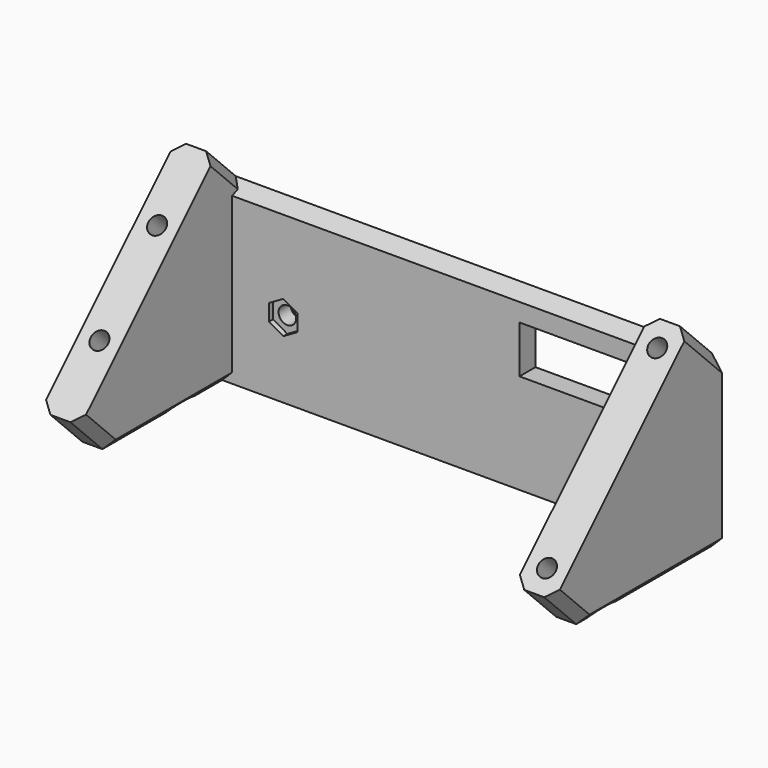
from build123d import *

# Parameters (mm, degrees)
F2_DEPTH      = 4
F5_DEPTH      = 49.55
F5_DEPTH_BACK = 53.25
F6_R          = 3.25
F6_R_2        = 1.75
F7_DEPTH      = 35.314708499
F8_DEPTH      = 5
F9_R          = 1.75
F9_W          = 23
F9_H          = 9.5
F10_DEPTH     = 4.001
F11_DEPTH     = 1
F12_T1_DEPTH  = 21.6004404508
F12_T3_DEPTH  = 86.8
F12_T5_DEPTH  = 21.6004404508
F12_T7_DEPTH  = 44.2278574488
F12_T9_DEPTH  = 35.0844914729
F12_T14_DEPTH = 15.9435862014
F12_T19_DEPTH = 15.9435862014
F12_T25_DEPTH = 98.9490097203
F12_S28_R     = 3.25
F12_T29_DEPTH = 51
F12_T32_DEPTH = 10.8002202254
F12_T39_DEPTH = 10.8002202254
F12_T43_DEPTH = 98.9490097203


# Not quite as in the source:
# - a fillet or chamfer that OpenCascade refuses, or shapes differently, is made with other operations: its cross-section is extruded or revolved along the edge and cut away or added


with BuildPart() as f2:
    # F0 (on Right) → F2 (new body, symmetric)
    with BuildSketch(Plane.YZ):
        Polygon((-8, 41.941125497), (-24.9705627485, 24.9705627485), (-41.941125497, 8), (-33.941125497, 0), (-4, 0), (-4, 37.941125497), align=None)
    extrude(amount=F2_DEPTH, both=True)


with BuildPart() as f3_1:
    # F3: copy of F2
    add(f2.part.moved(Location((-49.25, 0, 0))))


with BuildPart() as f2_1:
    # F4: moved
    add(f2.part.moved(Location((45.55, 0, 0))))


    add(f3_1.part)  # F5 merges F3_1
    # F0 (on Right) → F5 (join, two sides)
    with BuildSketch(Plane.YZ) as f5_sk:
        Polygon((0, 33.941125497), (-4, 37.941125497), (-4, 0), (0, 0), align=None)
    extrude(amount=F5_DEPTH)
    extrude(f5_sk.sketch, amount=-F5_DEPTH_BACK)

    # F6 (on line) → F7 (cut, through all)
    with BuildSketch(Plane(origin=(0, -24.9705627485, 24.9705627485), x_dir=(1, 0, 0), z_dir=(0, -0.7071067812, 0.7071067812))):
        with Locations((-49.25, 10.2)):
            Circle(F6_R)
        with Locations((-49.25, 10.2)):
            Circle(F6_R_2, mode=Mode.SUBTRACT)
        with Locations((-49.25, 10.2)):
            Circle(F6_R_2)
        with Locations((-49.25, -10.2)):
            Circle(F6_R)
        with Locations((-49.25, -10.2)):
            Circle(F6_R_2, mode=Mode.SUBTRACT)
        with Locations((-49.25, -10.2)):
            Circle(F6_R_2)
        with Locations((45.55, 19.5)):
            Circle(F6_R)
        with Locations((45.55, 19.5)):
            Circle(F6_R_2, mode=Mode.SUBTRACT)
        with Locations((45.55, 19.5)):
            Circle(F6_R_2)
        with Locations((45.55, -19.5)):
            Circle(F6_R)
        with Locations((45.55, -19.5)):
            Circle(F6_R_2, mode=Mode.SUBTRACT)
        with Locations((45.55, -19.5)):
            Circle(F6_R_2)
    extrude(amount=-F7_DEPTH, mode=Mode.SUBTRACT)

    # F6 (on line) → F8 (join)
    with BuildSketch(Plane(origin=(0, -24.9705627485, 24.9705627485), x_dir=(1, 0, 0), z_dir=(0, -0.7071067812, 0.7071067812))):
        with Locations((45.55, -19.5)):
            Circle(F6_R)
        with Locations((45.55, -19.5)):
            Circle(F6_R_2, mode=Mode.SUBTRACT)
        with Locations((45.55, 19.5)):
            Circle(F6_R)
        with Locations((45.55, 19.5)):
            Circle(F6_R_2, mode=Mode.SUBTRACT)
        with Locations((-49.25, 10.2)):
            Circle(F6_R)
        with Locations((-49.25, 10.2)):
            Circle(F6_R_2, mode=Mode.SUBTRACT)
        with Locations((-49.25, -10.2)):
            Circle(F6_R)
        with Locations((-49.25, -10.2)):
            Circle(F6_R_2, mode=Mode.SUBTRACT)
    extrude(amount=-F8_DEPTH)

    # F9 (on face) → F10 (cut, through all)
    with BuildSketch(Plane.XZ.offset(4)):
        with Locations((-35, 15)):
            Circle(F9_R)
        with Locations((35, 15)):
            Circle(F9_R)
        with Locations((23.75, 24.75)):
            Rectangle(F9_W, F9_H)
    extrude(amount=-F10_DEPTH, mode=Mode.SUBTRACT)

    # F9 (on face) → F11 (cut)
    with BuildSketch(Plane.XZ.offset(4)):
        Polygon((-32.15, 13.3545517328), (-32.15, 16.6454482672), (-35, 18.2908965344), (-37.85, 16.6454482672), (-37.85, 13.3545517328), (-35, 11.7091034656), align=None)
        with Locations((-35, 15)):
            Circle(F9_R, mode=Mode.SUBTRACT)
        Polygon((37.85, 13.3545517328), (37.85, 16.6454482672), (35, 18.2908965344), (32.15, 16.6454482672), (32.15, 13.3545517328), (35, 11.7091034656), align=None)
        with Locations((35, 15)):
            Circle(F9_R, mode=Mode.SUBTRACT)
    extrude(amount=-F11_DEPTH, mode=Mode.SUBTRACT)

    # F12: chamfer of 2 on 13 edges, made by hand

    # F12_s2 → F12_t1 (cut)
    with BuildSketch(Plane(origin=(0, -28.6074717082, 28.6074717082), x_dir=(1, 0, 0), z_dir=(0, 0.7071067812, -0.7071067812))):
        Polygon((47.55, -24), (49.55, -22), (49.55, -24), align=None)
        Polygon((-53.25, 22), (-51.25, 24), (-53.25, 24), align=None)
        Polygon((-45.25, 22), (-47.25, 24), (-45.25, 24), align=None)
        Polygon((41.55, 22), (43.55, 24), (41.55, 24), align=None)
        Polygon((49.55, 22), (47.55, 24), (49.55, 24), align=None)
    extrude(amount=F12_T1_DEPTH, mode=Mode.SUBTRACT)

    # F12_s4 → F12_t3 (cut)
    with BuildSketch(Plane.YZ.offset(-45.25)):
        Polygon((-0.5857864376, 34.5269119346), (-4, 33.1126983722), (-4, 37.941125497), align=None)
    extrude(amount=F12_T3_DEPTH, mode=Mode.SUBTRACT)

    # F12_s6 → F12_t5 (cut)
    with BuildSketch(Plane(origin=(0, -13.3336537888, 13.3336537888), x_dir=(1, 0, 0), z_dir=(0, -0.7071067812, 0.7071067812))):
        Polygon((-51.25, 24), (-53.25, 22), (-53.25, 24), align=None)
    extrude(amount=F12_T5_DEPTH, mode=Mode.SUBTRACT)

    # F12_s8 → F12_t7 (cut)
    with BuildSketch(Plane.XZ.offset(-5.1433659759)):
        Polygon((-53.25, 2), (-51.25, 0), (-53.25, 0), align=None)
        Polygon((49.55, 2), (47.55, 0), (49.55, 0), align=None)
    extrude(amount=F12_T7_DEPTH, mode=Mode.SUBTRACT)

    # F12_s10 → F12_t9 (cut)
    with BuildSketch(Plane.XZ.offset(4)):
        Polygon((-45.25, 2), (-47.25, 0), (-45.25, 0), align=None)
        Polygon((41.55, 2), (43.55, 0), (41.55, 0), align=None)
    extrude(amount=F12_T9_DEPTH, mode=Mode.SUBTRACT)


with BuildPart() as f12_tool12:
    # F12_s13 → F12_t14 (new body)
    with BuildSketch(Plane(origin=(0, -17.3336537888, 17.3336537888), x_dir=(1, 0, 0), z_dir=(0, -0.7071067812, 0.7071067812))):
        Polygon((-47.25, 24), (-45.25, 22), (-45.25, 24), align=None)
    extrude(amount=F12_T14_DEPTH)

    split(bisect_by=Plane.XZ.offset(4), keep=Keep.TOP)


with BuildPart() as f2_2:
    add(f2_1.part)

    # F12_t11: cut F12_tool12
    add(f12_tool12.part, mode=Mode.SUBTRACT)


with BuildPart() as f12_tool17:
    # F12_s18 → F12_t19 (new body)
    with BuildSketch(Plane(origin=(0, -17.3336537888, 17.3336537888), x_dir=(1, 0, 0), z_dir=(0, -0.7071067812, 0.7071067812))):
        Polygon((43.55, 24), (41.55, 22), (41.55, 24), align=None)
    extrude(amount=F12_T19_DEPTH)

    split(bisect_by=Plane.XZ.offset(4), keep=Keep.TOP)


with BuildPart() as f2_3:
    add(f2_2.part)

    # F12_t16: cut F12_tool17
    add(f12_tool17.part, mode=Mode.SUBTRACT)


with BuildPart() as f12_tool23:
    # F12_s24 → F12_t25 (new body)
    with BuildSketch(Plane.YZ.offset(53.6990097203)):
        Polygon((-0.5857864376, 34.5269119346), (-4, 33.1126983722), (-4, 37.941125497), align=None)
    extrude(amount=-F12_T25_DEPTH)

    split(bisect_by=Plane.YZ.offset(41.55), keep=Keep.TOP)

    split(bisect_by=Plane.YZ.offset(49.55), keep=Keep.BOTTOM)

    # F12_s28 → F12_t29 (cut, symmetric)
    with BuildSketch(Plane(origin=(0, -18.8797510577, 18.8797510577), x_dir=(1, 0, 0), z_dir=(0, -0.7071067812, 0.7071067812))):
        with Locations((45.55, 19.5)):
            Circle(F12_S28_R)
    extrude(amount=F12_T29_DEPTH, both=True, mode=Mode.SUBTRACT)


with BuildPart() as f12_tool30:
    # F12_s31 → F12_t32 (new body)
    with BuildSketch(Plane(origin=(0, -17.3336537888, 17.3336537888), x_dir=(1, 0, 0), z_dir=(0, -0.7071067812, 0.7071067812))):
        Polygon((43.55, 24), (41.55, 22), (41.55, 24), align=None)
    extrude(amount=F12_T32_DEPTH)

    split(bisect_by=Plane.XZ.offset(4), keep=Keep.BOTTOM)


with BuildPart() as f12_tool23_1:
    add(f12_tool23.part)

    # F12_t34: intersect F12_tool30
    add(f12_tool30.part, mode=Mode.INTERSECT)


with BuildPart() as f2_4:
    add(f2_3.part)

    # F12_t21: cut F12_tool23
    add(f12_tool23_1.part, mode=Mode.SUBTRACT)


with BuildPart() as f12_tool37:
    # F12_s38 → F12_t39 (new body)
    with BuildSketch(Plane(origin=(0, -17.3336537888, 17.3336537888), x_dir=(1, 0, 0), z_dir=(0, -0.7071067812, 0.7071067812))):
        Polygon((-47.25, 24), (-45.25, 22), (-45.25, 24), align=None)
    extrude(amount=F12_T39_DEPTH)

    split(bisect_by=Plane.XZ.offset(4), keep=Keep.BOTTOM)


with BuildPart() as f12_tool41:
    # F12_s42 → F12_t43 (new body)
    with BuildSketch(Plane.YZ.offset(41.55)):
        Polygon((-0.5857864376, 34.5269119346), (-4, 33.1126983722), (-4, 37.941125497), align=None)
    extrude(amount=-F12_T43_DEPTH)

    split(bisect_by=Plane.YZ.offset(-45.25), keep=Keep.BOTTOM)

    split(bisect_by=Plane.YZ.offset(-53.25), keep=Keep.TOP)


with BuildPart() as f12_tool37_1:
    add(f12_tool37.part)

    # F12_t46: intersect F12_tool41
    add(f12_tool41.part, mode=Mode.INTERSECT)


with BuildPart() as f2_5:
    add(f2_4.part)

    # F12_t35: cut F12_tool37
    add(f12_tool37_1.part, mode=Mode.SUBTRACT)


solid = f2_5.part
